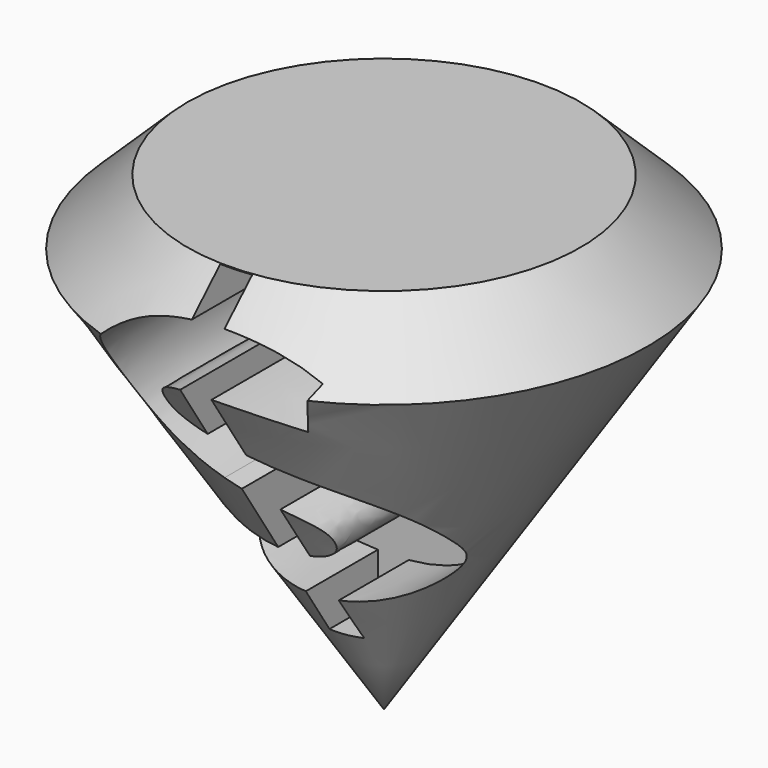
from build123d import *

# Parameters (mm, degrees)
F2_TEXT_SIZE = 110.0002581047
F3_DEPTH     = 86.614


# Not quite as in the source:
# - Text() gives the source's letters only with a copy of the font that has no kerning and outlines rounded to 1/6400 em; it was checked with that copy


with BuildPart() as f1:
    # F0 (on Front) → F1 (revolve)
    with BuildSketch(Plane.XZ):
        Polygon((0, 55.9584125876), (-46.8884520233, 55.9584125876), (-62.9228428006, 40.4099114239), (0, -56.2823414803), align=None)
    revolve(axis=Axis((0, 0, -0.1619644463), (0, 0, -1)))

    # F2 (on Front) → F3 (cut)
    with BuildSketch(Plane.XZ):
        with Locations((-29.2866842938, -27.6134070009)):
            Text('$', F2_TEXT_SIZE, font='Open Sans', font_style=FontStyle.BOLD, text_align=(TextAlign.LEFT, TextAlign.BOTTOM))
    extrude(amount=F3_DEPTH, mode=Mode.SUBTRACT)


solid = f1.part
